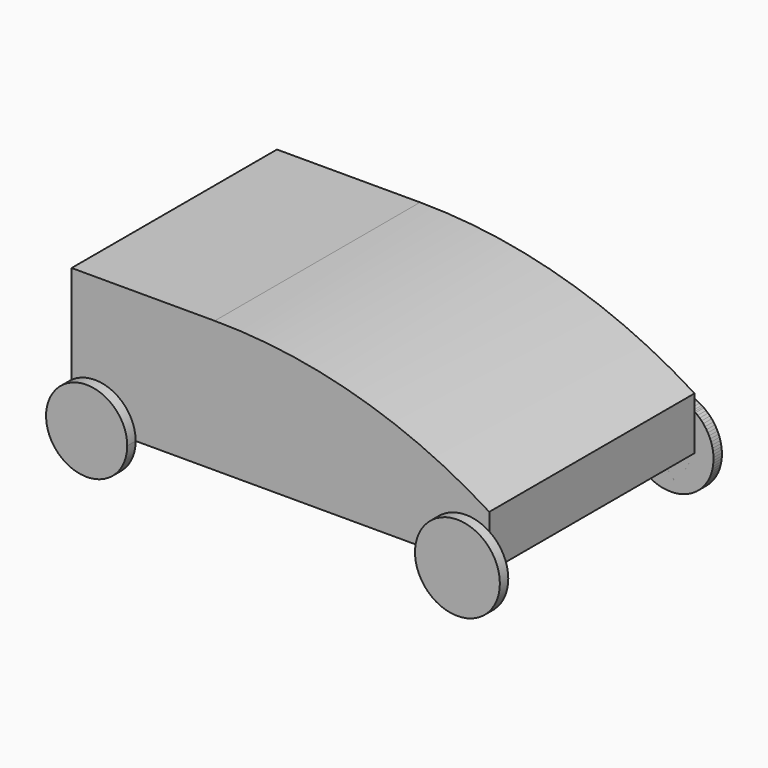
from build123d import *

# Parameters (mm, degrees)
F0_W         = 79.3992951512
F0_H         = 48.7897545099
F1_DEPTH     = 20
F3_DEPTH     = 2
F2_R         = 7.716624038
F2_R_2       = 8.0676554741
F4_DEPTH     = 2
F5_DEPTH     = 25
F7_DEPTH     = 2
F6_R         = 8.1319120556
F8_DEPTH     = 2
F6_R_2       = 7.3501994426
F9_SIZE      = 15
F10_T1_DEPTH = 234.764288605


# Not quite as in the source:
# - a fillet or chamfer that OpenCascade refuses, or shapes differently, is made with other operations: its cross-section is extruded or revolved along the edge and cut away or added


with BuildPart() as f1:
    # F0 (on Top) → F1 (new body)
    with BuildSketch(Plane.XY):
        Rectangle(F0_W, F0_H)
    extrude(amount=F1_DEPTH)

    # F2 (on face) → F3 (join)
    with BuildSketch(Plane.XZ.offset(24.394877255)):
        with BuildLine():
            ThreePointArc((-39.6996475756, 6.3026463031), (-38.7962669692, -6.8521156516), (-27.5307279362, 0))
            Line((-27.5307279362, 0), (-39.6996475756, 0))
            Line((-39.6996475756, 0), (-39.6996475756, 6.3026463031))
        make_face()
        with BuildLine():
            Line((-39.6996475756, 0), (-27.5307279362, 0))
            ThreePointArc((-27.5307279362, 0), (-31.6984369793, 6.8521156516), (-39.6996475756, 6.3026463031))
            Line((-39.6996475756, 6.3026463031), (-39.6996475756, 0))
        make_face()
    extrude(amount=F3_DEPTH)

    # F2 (on face) → F4 (join)
    with BuildSketch(Plane.XZ.offset(24.394877255)):
        with Locations((-35.2473519742, 0)):
            Circle(F2_R)
        with Locations((35.2473519742, 0)):
            Circle(F2_R_2)
    extrude(amount=F4_DEPTH)

    # F5 (add): a face of the model
    f5_faces = [f1.faces().sort_by_distance(p)[0] for p in [
        (0, 0, 0),
    ]]
    extrude(f5_faces, amount=-F5_DEPTH)

    # F6 (on face) → F7 (join)
    with BuildSketch(Plane(origin=(0, 24.394877255, 0), x_dir=(-1, 0, 0), z_dir=(0, 1, 0))):
        with BuildLine():
            Line((-39.6996475756, 0), (-39.6996475756, 6.9567142054))
            ThreePointArc((-39.6996475756, 6.9567142054), (-39.085462227, -6.9230727989), (-27.0398499989, 0))
            Line((-27.0398499989, 0), (-39.6996475756, 0))
        make_face()
        with BuildLine():
            ThreePointArc((-27.0398499989, 0), (-27.0379361612, 0.1018445872), (-27.0372981819, 0.2037051572))
            ThreePointArc((-27.0372981819, 0.2037051572), (-31.3425357234, 7.3789790783), (-39.6996475756, 6.9567142054))
            Line((-39.6996475756, 6.9567142054), (-39.6996475756, 0))
            Line((-39.6996475756, 0), (-27.0398499989, 0))
        make_face()
        with BuildLine():
            Line((39.6996475756, 0), (28.2432777683, 0))
            ThreePointArc((28.2432777683, 0), (35.7958396069, -6.9173753491), (42.9311066746, 0.4296809267))
            ThreePointArc((42.9311066746, 0.4296809267), (42.0731716607, 3.875828694), (39.6996475756, 6.517489221))
            Line((39.6996475756, 6.517489221), (39.6996475756, 0))
        make_face()
    extrude(amount=F7_DEPTH)

    # F9
    f9_edges = [f1.edges().sort_by_distance(p)[0] for p in [
        (39.699648, 0, 25),
    ]]
    chamfer(f9_edges, length=F9_SIZE)

    # F10: fillet of radius 98.3102765948 on 1 edges, made by hand

    # F10_s2 → F10_t1 (cut)
    with BuildSketch(Plane.XZ.offset(-117.3821443025)):
        with BuildLine():
            ThreePointArc((-12.4952592434, 25), (14.6585079807, 21.1756134083), (39.6996475756, 10))
            Line((39.6996475756, 10), (24.6996475756, 25))
            Line((24.6996475756, 25), (-12.4952592434, 25))
        make_face()
    extrude(amount=F10_T1_DEPTH, mode=Mode.SUBTRACT)


with BuildPart() as f8:
    # F6 (on face) → F8 (new body)
    with BuildSketch(Plane(origin=(0, 24.394877255, 0), x_dir=(-1, 0, 0), z_dir=(0, 1, 0))):
        with Locations((-35.1692102375, 0.2037051572)):
            Circle(F6_R)
    extrude(amount=F8_DEPTH)


with BuildPart() as f8b:
    # F6 (on face) → F8, piece 2 (new body)
    with BuildSketch(Plane(origin=(0, 24.394877255, 0), x_dir=(-1, 0, 0), z_dir=(0, 1, 0))):
        with Locations((35.580907232, 0.4296809267)):
            Circle(F6_R_2)
    extrude(amount=F8_DEPTH)


solid = Compound([f1.part, f8.part, f8b.part])
